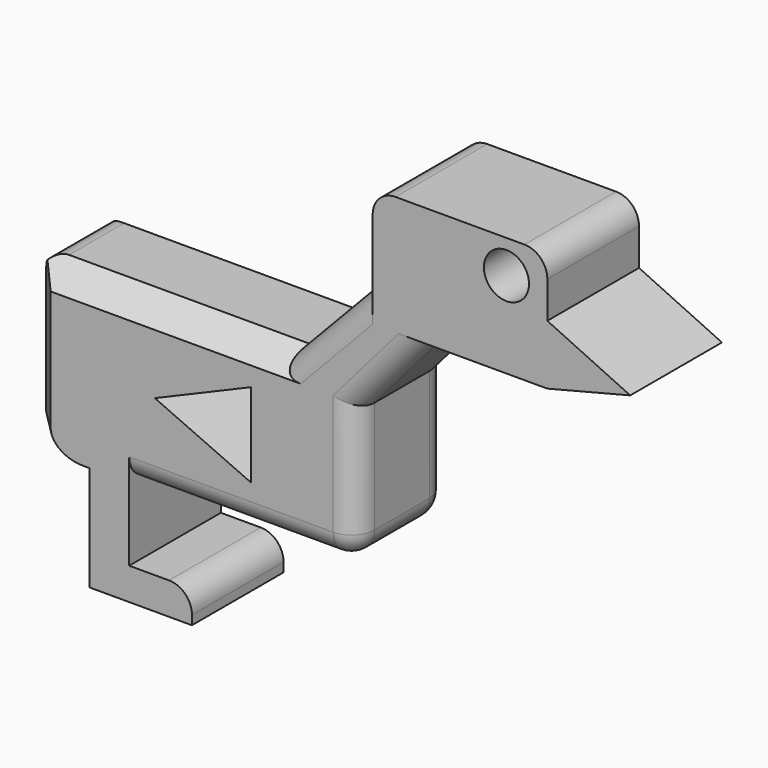
from build123d import *

# Parameters (mm, degrees)
F0_R     = 4.998133971
F1_DEPTH = 25.4
F2_R     = 5.08
F3_SIZE  = 5.08
F4_SIZE  = 5.08
F5_R     = 5.08
F6_R     = 5.08
F7_R     = 5.08
F8_R     = 5.08
F9_R     = 5.08


with BuildPart() as f1:
    # F0 (on Front) → F1 (new body)
    with BuildSketch(Plane.XZ):
        Polygon((-13.9009580016, -18.3790195733), (36.3904610276, -18.3790195733), (36.3904610276, 11.5175191313), (36.3904610276, 18.3790195733), (21.9322983176, 18.3790195733), (-36.3904610276, 18.3790195733), (-36.3904610276, -18.3790195733), (-22.7228868753, -18.3790195733), (-22.7228868753, -41.6591130197), (0, -41.6591130197), (0, -34.5525592566), (-13.9009580016, -34.5525592566), align=None)
        Polygon((-8.2092965022, 0), (13.1103685126, 9.0669831261), (13.1103685126, -9.5570906997), align=None, mode=Mode.SUBTRACT)
        Polygon((36.3904610276, 18.3790195733), (36.3904610276, 11.5175191313), (52.5639988482, 30.1415920258), (78.7847340107, 30.1415920258), (78.7847340107, 43.3744862676), (78.7847340107, 56.6073805094), (40.0662571192, 56.6073805094), (40.0662571192, 37.4673998365), (21.9322983176, 18.3790195733), align=None)
        with Locations((69.7177499533, 49.2557734251)):
            Circle(F0_R, mode=Mode.SUBTRACT)
        Polygon((78.7847340107, 43.3744862676), (78.7847340107, 30.1415920258), (97.1637517214, 34.7976125777), align=None)
    extrude(amount=F1_DEPTH)

    # F2
    f2_edges = [f1.edges().sort_by_distance(p)[0] for p in [
        (0, -12.7, -34.552559),
    ]]
    fillet(f2_edges, radius=F2_R)

    # F3
    f3_edges = [f1.edges().sort_by_distance(p)[0] for p in [
        (-7.229081, -25.4, 18.37902),
        (-36.390461, -25.4, 0),
    ]]
    chamfer(f3_edges, length=F3_SIZE)

    # F4
    f4_edges = [f1.edges().sort_by_distance(p)[0] for p in [
        (-7.229081, 0, 18.37902),
        (-36.390461, 0, 0),
    ]]
    chamfer(f4_edges, length=F4_SIZE)

    # F5
    f5_edges = [f1.edges().sort_by_distance(p)[0] for p in [
        (-36.390461, -12.7, 18.37902),
    ]]
    fillet(f5_edges, radius=F5_R)

    # F6
    f6_edges = [f1.edges().sort_by_distance(p)[0] for p in [
        (78.784734, -12.7, 56.607381),
        (40.066257, -12.7, 56.607381),
    ]]
    fillet(f6_edges, radius=F6_R)

    # F7
    f7_edges = [f1.edges().sort_by_distance(p)[0] for p in [
        (36.390461, -12.7, -18.37902),
    ]]
    fillet(f7_edges, radius=F7_R)

    # F8
    f8_edges = [f1.edges().sort_by_distance(p)[0] for p in [
        (-36.390461, -12.7, -18.37902),
        (-33.850461, -22.86, -18.37902),
        (-33.850461, -2.54, -18.37902),
    ]]
    fillet(f8_edges, radius=F8_R)

    # F9
    f9_edges = [f1.edges().sort_by_distance(p)[0] for p in [
        (30.999278, -25.4, 27.92321),
        (30.999278, 0, 27.92321),
        (44.47723, -25.4, 20.829556),
        (36.390461, -25.4, -0.89075),
        (44.47723, 0, 20.829556),
        (36.390461, 0, -0.89075),
    ]]
    fillet(f9_edges, radius=F9_R)


solid = f1.part
